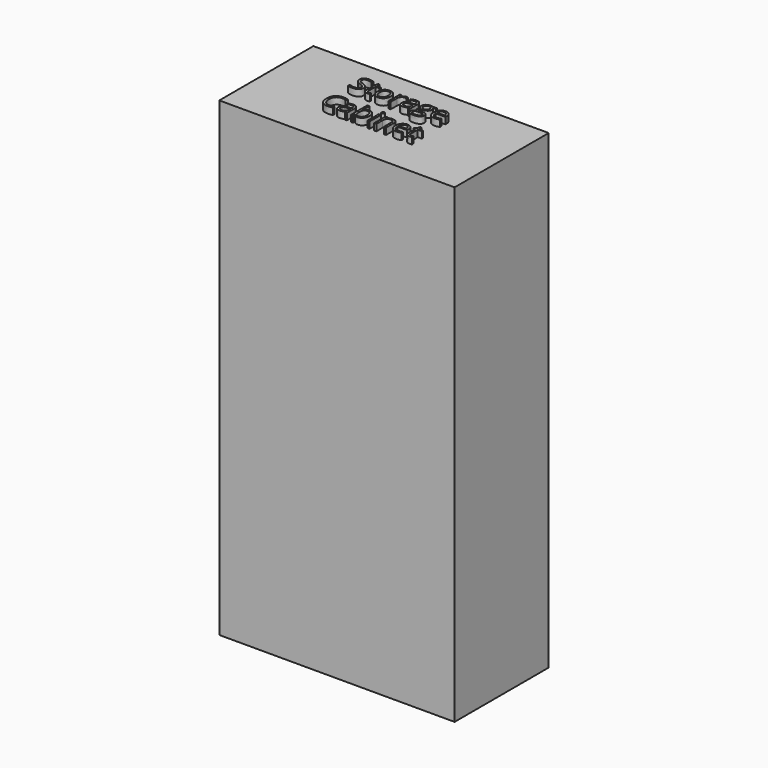
from build123d import *

# Parameters (mm, degrees)
F0_W         = 914.4
F0_H         = 457.2
F1_DEPTH     = 1828.8
F2_TEXT_SIZE = 103.1705747462
F3_DEPTH     = 25.4


# Not quite as in the source:
# - Text() gives the source's letters only with a copy of the font that has no kerning and outlines rounded to 1/6400 em; it was checked with that copy


with BuildPart() as f1:
    # F0 (on Top) → F1 (new body)
    with BuildSketch(Plane.XY):
        Rectangle(F0_W, F0_H)
    extrude(amount=F1_DEPTH)

    # F2 (on face) → F3 (join)
    with BuildSketch(Plane.XY.offset(1828.8)):
        with Locations((-186.972486124, 50.5827255547)):
            Text('Storage', F2_TEXT_SIZE, font='Open Sans', text_align=(TextAlign.LEFT, TextAlign.BOTTOM))
        with Locations((-186.972486124, -89.7292561001)):
            Text('Cabinet', F2_TEXT_SIZE, font='Open Sans', text_align=(TextAlign.LEFT, TextAlign.BOTTOM))
    extrude(amount=F3_DEPTH)


solid = f1.part
